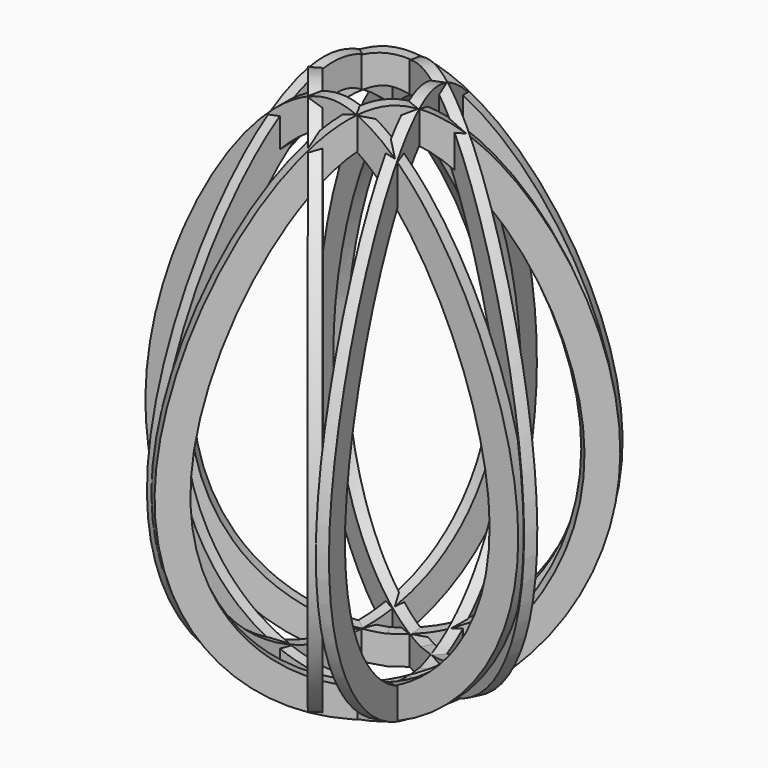
from build123d import *

# Parameters (mm, degrees)
F2_DEPTH = 2.54
F4_COUNT = 7


# Not quite as in the source:
# - the dataset's text gives a spline's control points without its knots; the knots are read off the source's solid


with BuildPart() as f2:
    # F1 (on offset) → F2 (new body)
    with BuildSketch(Plane.XZ.offset(8.89)):
        with BuildLine():
            add(Edge.make_bspline(
                [(0, 61.3641925156), (17.4292388531, 61.3641925156), (61.6951390769, -14.5327890586), (23.980735402, -57.4269294555), (0, -58.3029389381)],
                knots=[0, 0, 0, 0, 0.532927507, 1, 1, 1, 1], degree=3))
            add(Edge.make_bspline(
                [(0, 61.3641925156), (-17.4292388531, 61.3641925156), (-61.6951390769, -14.5327890586), (-23.980735402, -57.4269294555), (0, -58.3029389381)],
                knots=[0, 0, 0, 0, 0.532927507, 1, 1, 1, 1], degree=3))
        make_face()
        with BuildLine():
            add(Edge.make_bspline(
                [(0, 55.0141925156), (-0.445947753, 55.0141925156), (-1.4791581814, 54.8946082931), (-3.5407762672, 54.1560645792), (-5.9999081331, 52.7409173772), (-8.7151023729, 50.6426655614), (-11.5703509862, 47.9054441805), (-15.4466505436, 43.4887139916), (-20.2438132358, 36.7027631623), (-25.4948344209, 27.0937270461), (-29.8985850611, 16.566633738), (-32.6059034429, 7.4849258878), (-34.0569829874, 0.3153056303), (-34.6412328524, -4.0646979957), (-34.9021143227, -7.4714967382), (-34.9920055804, -9.9669999406), (-34.9737708348, -12.3997980071), (-34.8091353058, -15.5745360602), (-34.3481094285, -19.4007161053), (-33.098373903, -25.2009442296), (-30.6361061969, -31.8076865533), (-26.4250321863, -38.5910042258), (-21.125050611, -44.1262594423), (-14.875830381, -48.3192642683), (-7.8439260979, -51.0448266213), (-2.6676745415, -51.8343431277), (0, -51.9479999425)],
                knots=[0, 0, 0, 0, 0.03125, 0.0625, 0.09375, 0.125, 0.15625, 0.1875, 0.25, 0.3125, 0.375, 0.4375, 0.46875, 0.5, 0.515625, 0.53125, 0.546875, 0.5625, 0.59375, 0.625, 0.6875, 0.75, 0.8125, 0.875, 0.9375, 0.9982427912, 0.9982427912, 0.9982427912, 0.9982427912], degree=3))
            add(Edge.make_bspline(
                [(0, 55.0141925156), (0.445947753, 55.0141925156), (1.4791581814, 54.8946082931), (3.5407762672, 54.1560645792), (5.9999081331, 52.7409173772), (8.7151023729, 50.6426655614), (11.5703509862, 47.9054441805), (15.4466505436, 43.4887139916), (20.2438132358, 36.7027631623), (25.4948344209, 27.0937270461), (29.8985850611, 16.566633738), (32.6059034429, 7.4849258878), (34.0569829874, 0.3153056303), (34.6412328524, -4.0646979957), (34.9021143227, -7.4714967382), (34.9920055804, -9.9669999406), (34.9737708348, -12.3997980071), (34.8091353058, -15.5745360602), (34.3481094285, -19.4007161053), (33.098373903, -25.2009442296), (30.6361061969, -31.8076865533), (26.4250321863, -38.5910042258), (21.125050611, -44.1262594423), (14.875830381, -48.3192642683), (7.8439260979, -51.0448266213), (2.6676745415, -51.8343431277), (0, -51.9479999425)],
                knots=[0, 0, 0, 0, 0.03125, 0.0625, 0.09375, 0.125, 0.15625, 0.1875, 0.25, 0.3125, 0.375, 0.4375, 0.46875, 0.5, 0.515625, 0.53125, 0.546875, 0.5625, 0.59375, 0.625, 0.6875, 0.75, 0.8125, 0.875, 0.9375, 0.9982427912, 0.9982427912, 0.9982427912, 0.9982427912], degree=3))
        make_face(mode=Mode.SUBTRACT)
    extrude(amount=F2_DEPTH)

    # F4: F2 ×7 about axis
    f4_axis = Axis((0.2033080673, 0, 39.8002751172), (0, 0, 1))


with BuildPart() as f2_1:
    add(f2.part)
    for i in range(1, F4_COUNT):
        add(f2.part.rotate(f4_axis, i * 360 / F4_COUNT))


solid = f2_1.part
